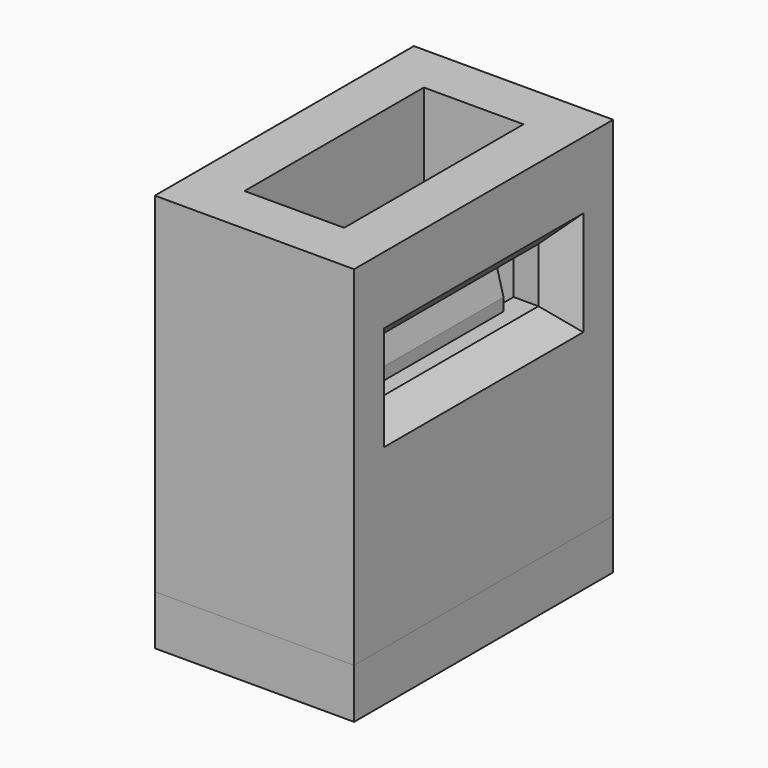
from build123d import *

# Parameters (mm, degrees)
F0_W          = 8
F0_H          = 13
F1_DEPTH      = 14
F3_W          = 8
F3_H          = 13
F3_W_2        = 4
F3_H_2        = 9
F3_W_3        = 2.8
F3_H_3        = 7.8
F4_DEPTH      = 2
F5_DEPTH      = 1
F6_DEPTH      = 3
F6_DEPTH_BACK = 3
F7_R          = 0.5
F8_DEPTH      = 4
F8_DEPTH_BACK = 4
F9_SIZE       = 1


with BuildPart() as f1:
    # F0 (on Top) → F1 (new body)
    with BuildSketch(Plane.XY):
        Rectangle(F0_W, F0_H)
        Polygon((-2, 0), (-2, 4.5), (0, 4.5), (2, 4.5), (2, 0), (2, -4.5), (0, -4.5), (-2, -4.5), align=None, mode=Mode.SUBTRACT)
    extrude(amount=F1_DEPTH)

    # F2 (on Front) → F8 (cut, two sides)
    with BuildSketch(Plane.XZ) as f8_sk:
        Polygon((2, 10.3), (2, 10), (2.03134729, 10), (2.4, 10), (2.4, 8.6241693561), (2.4, 8.1241693561), (2.4, 8.0991693561), (5.4, 8.0991693561), (5.4, 10.3), align=None)
        Polygon((-1.5, 8.0991693561), (-1.4, 8.0991693561), (-1.4, 10), (-0.8759222072, 10), (2, 10), (2, 10.3), (-1.5, 10.3), align=None)
        Polygon((-1.4, 8.0991693561), (-0.97554052, 8.0991693561), (-0.8759222072, 10), (-1.4, 10), align=None)
        Polygon((2.4, 10), (2.03134729, 10), (2.4, 8.6241693561), align=None)
        Polygon((-0.8759222072, 10), (-0.97554052, 8.0991693561), (2, 8.0991693561), (2, 10), align=None)
        Polygon((2, 10), (2, 8.0991693561), (2.1142486924, 8.0991693561), (2.4, 8.1241693561), (2.4, 8.6241693561), (2.03134729, 10), align=None)
        Polygon((2.4, 8.1241693561), (2.1142486924, 8.0991693561), (2.4, 8.0991693561), align=None)
    extrude(amount=-F8_DEPTH, mode=Mode.SUBTRACT)
    extrude(f8_sk.sketch, amount=F8_DEPTH_BACK, mode=Mode.SUBTRACT)

    # F9
    f9_edges = [f1.edges().sort_by_distance(p)[0] for p in [
        (4, 0, 10.3),
        (4, 4, 9.199585),
        (4, 0, 8.099169),
        (4, -4, 9.199585),
    ]]
    chamfer(f9_edges, length=F9_SIZE)


with BuildPart() as f4:
    # F3 (on face) → F4 (new body)
    with BuildSketch(Plane(origin=(0, 0, 0), x_dir=(1, 0, 0), z_dir=(0, 0, -1))):
        Rectangle(F3_W, F3_H)
        Rectangle(F3_W_2, F3_H_2, mode=Mode.SUBTRACT)
        Rectangle(F3_W_2, F3_H_2)
        Polygon((-1.9, 3.9), (-1.9, 4.4), (1.9, 4.4), (1.9, -4.4), (-1.9, -4.4), (-1.9, -3.9), align=None, mode=Mode.SUBTRACT)
        with Locations((-0.5, 0)):
            Rectangle(F3_W_3, F3_H_3)
        Polygon((1.9, 4.4), (-1.9, 4.4), (-1.9, 3.9), (0.9, 3.9), (0.9, -3.9), (-1.9, -3.9), (-1.9, -4.4), (1.9, -4.4), align=None)
    extrude(amount=F4_DEPTH)

    # F3 (on face) → F5 (join)
    with BuildSketch(Plane(origin=(0, 0, 0), x_dir=(1, 0, 0), z_dir=(0, 0, -1))):
        Polygon((1.9, 4.4), (-1.9, 4.4), (-1.9, 3.9), (0.9, 3.9), (0.9, -3.9), (-1.9, -3.9), (-1.9, -4.4), (1.9, -4.4), align=None)
    extrude(amount=-F5_DEPTH)

    # F2 (on Front) → F6 (join, two sides)
    with BuildSketch(Plane.XZ) as f6_sk:
        Polygon((-0.97554052, 8.0991693561), (-1.4, 0), (1.4, 0), (0.9807377657, 8), (2, 8.0891738907), (2, 8.0991693561), align=None)
        Polygon((2, 10), (2, 8.0991693561), (2.1142486924, 8.0991693561), (2.4, 8.1241693561), (2.4, 8.6241693561), (2.03134729, 10), align=None)
        Polygon((-0.8759222072, 10), (-0.97554052, 8.0991693561), (2, 8.0991693561), (2, 10), align=None)
    extrude(amount=F6_DEPTH)
    extrude(f6_sk.sketch, amount=-F6_DEPTH_BACK)

    # F7
    f7_edges = [f4.edges().sort_by_distance(p)[0] for p in [
        (-1.4, 0, 0),
        (1.347592, 0, 1),
    ]]
    fillet(f7_edges, radius=F7_R)


solid = Compound([f1.part, f4.part])
